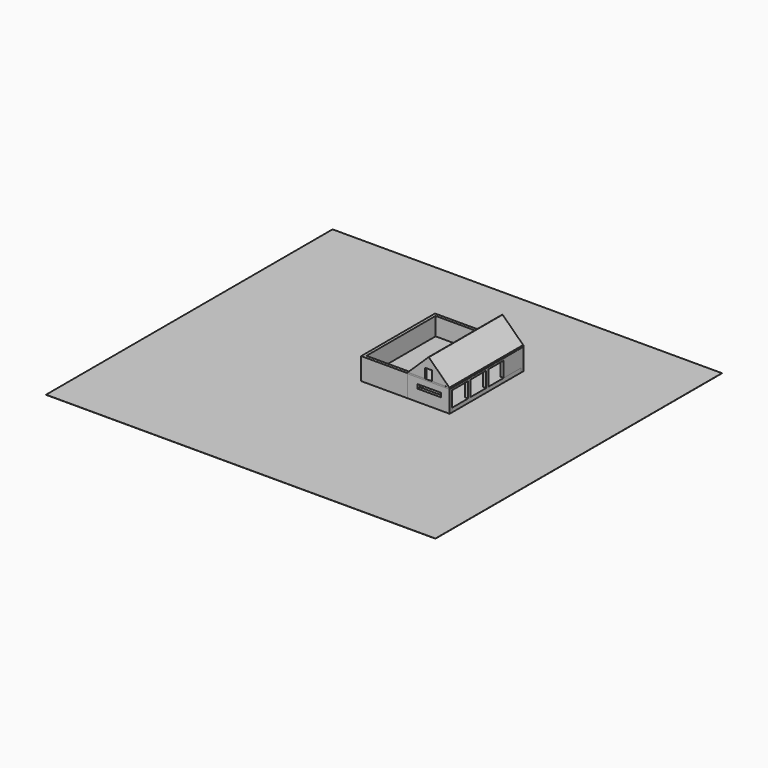
from build123d import *

# Parameters (mm, degrees)
F0_W      = 520
F0_H      = 3240
F0_H_2    = 520
F0_H_3    = 3380
F0_H_4    = 3450
F1_DEPTH  = 10
F2_DEPTH  = 3350
F3_W      = 520
F3_H      = 11110
F4_DEPTH  = 350
F5_W      = 7240
F5_H      = 200
F6_DEPTH  = 200
F7_W      = 7240
F7_H      = 15890
F8_DEPTH  = 3500
F9_SIZE2  = 3499.99999
F9_SIZE   = 3599.99999
F10_T     = 260
F11_W     = 1200
F11_H     = 1700
F12_DEPTH = 260
F13_W     = 6720
F13_H     = 14850
F14_DEPTH = 700
F15_W     = 7240
F15_H     = 15891
F16_DEPTH = 50
F17_W     = 1500
F17_H     = 2650
F18_DEPTH = 520
F19_W     = 4000
F19_H     = 700
F20_DEPTH = 520
F21_W     = 67073.4691619873
F21_H     = 61686.4318847656
F21_W_2   = 7240
F21_H_2   = 15890
F22_DEPTH = 25
F24_DEPTH = 3800
F25_W     = 7500
F25_H     = 14890
F26_DEPTH = 700


# Not quite as in the source:
# - a fillet or chamfer is up to 0.001 mm smaller than in the source, because OpenCascade refuses the exact size
# - a shell that OpenCascade refuses in one call is made with other operations: the cavity is built on its own and cut out
# - a feature names something its author has since deleted; it is built from what else it names


with BuildPart() as f1:
    # F0 (on Top) → F1 (new body)
    with BuildSketch(Plane.XY):
        Polygon((-3374.345998764, -8413.8299859681), (-3374.345998764, 6436.1700140319), (2825.654001236, 6436.1700140319), (2825.654001236, 2696.170014032), (3345.654001236, 2696.170014032), (3345.654001236, 6956.1700140319), (-3894.345998764, 6956.1700140319), (-3894.345998764, -8933.8299859681), (3345.654001236, -8933.8299859681), (3345.654001236, -8413.8299859681), (2825.654001236, -8413.8299859681), align=None)
        Polygon((2825.654001236, 6436.1700140319), (-3374.345998764, 6436.1700140319), (-3374.345998764, -8413.8299859681), (2825.654001236, -8413.8299859681), (2825.654001236, -4963.8299859681), (2825.654001236, -4443.829985968), (2825.654001236, -1063.8299859681), (2825.654001236, -543.829985968), (2825.654001236, 2696.170014032), align=None)
        with Locations((3085.654001236, 1076.170014032)):
            Rectangle(F0_W, F0_H)
        with Locations((3085.654001236, -803.829985968)):
            Rectangle(F0_W, F0_H_2)
        with Locations((3085.654001236, -2753.829985968)):
            Rectangle(F0_W, F0_H_3)
        with Locations((3085.654001236, -6688.8299859681)):
            Rectangle(F0_W, F0_H_4)
        with Locations((3085.654001236, -4703.8299859681)):
            Rectangle(F0_W, F0_H_2)
    extrude(amount=-F1_DEPTH)

    # F0 (on Top) → F2 (join)
    with BuildSketch(Plane.XY):
        with Locations((3085.654001236, -803.829985968)):
            Rectangle(F0_W, F0_H_2)
        with Locations((3085.654001236, -4703.8299859681)):
            Rectangle(F0_W, F0_H_2)
        Polygon((-3374.345998764, -8413.8299859681), (-3374.345998764, 6436.1700140319), (2825.654001236, 6436.1700140319), (2825.654001236, 2696.170014032), (3345.654001236, 2696.170014032), (3345.654001236, 6956.1700140319), (-3894.345998764, 6956.1700140319), (-3894.345998764, -8933.8299859681), (3345.654001236, -8933.8299859681), (3345.654001236, -8413.8299859681), (2825.654001236, -8413.8299859681), align=None)
    extrude(amount=F2_DEPTH)

    # F3 (on face) → F4 (join)
    with BuildSketch(Plane.XY.offset(3350)):
        Polygon((3345.654001236, 6956.1700140319), (-3894.345998764, 6956.1700140319), (-3894.345998764, -8933.8299859681), (3345.654001236, -8933.8299859681), (3345.654001236, -8413.8299859681), (2825.654001236, -8413.8299859681), (-3374.345998764, -8413.8299859681), (-3374.345998764, 6436.1700140319), (2825.654001236, 6436.1700140319), (2825.654001236, 2696.170014032), (3345.654001236, 2696.170014032), align=None)
        with Locations((3085.654001236, -2858.8299859681)):
            Rectangle(F3_W, F3_H)
    extrude(amount=F4_DEPTH)

    # F5 (on face) → F6 (join)
    with BuildSketch(Plane.XY.offset(3700)):
        with Locations((-274.345998764, 6856.1700140319)):
            Rectangle(F5_W, F5_H)
        with Locations((-274.345998764, 5649.1700140319)):
            Rectangle(F5_W, F5_H)
        with Locations((-274.345998764, 4442.1700140319)):
            Rectangle(F5_W, F5_H)
        with Locations((-274.345998764, 3235.1700140319)):
            Rectangle(F5_W, F5_H)
        with Locations((-274.345998764, 2028.1700140319)):
            Rectangle(F5_W, F5_H)
        with Locations((-274.345998764, 821.1700140319)):
            Rectangle(F5_W, F5_H)
        with Locations((-274.345998764, -385.8299859681)):
            Rectangle(F5_W, F5_H)
        with Locations((-274.345998764, -1592.8299859681)):
            Rectangle(F5_W, F5_H)
        with Locations((-274.345998764, -2799.8299859681)):
            Rectangle(F5_W, F5_H)
        with Locations((-274.345998764, -4006.8299859681)):
            Rectangle(F5_W, F5_H)
        with Locations((-274.345998764, -5213.8299859681)):
            Rectangle(F5_W, F5_H)
        with Locations((-274.345998764, -6420.8299859681)):
            Rectangle(F5_W, F5_H)
        with Locations((-274.345998764, -7627.8299859681)):
            Rectangle(F5_W, F5_H)
        with Locations((-274.345998764, -8834.8299859681)):
            Rectangle(F5_W, F5_H)
    extrude(amount=F6_DEPTH)

    # F17 (on face) → F18 (cut)
    with BuildSketch(Plane(origin=(-3894.345998764, 0, 0), x_dir=(0, -1, 0), z_dir=(-1, 0, 0))):
        with Locations((5683.8299859681, 2025)):
            Rectangle(F17_W, F17_H)
        with Locations((1683.8299859681, 2025)):
            Rectangle(F17_W, F17_H)
        with Locations((-2316.1700140319, 2025)):
            Rectangle(F17_W, F17_H)
    extrude(amount=-F18_DEPTH, mode=Mode.SUBTRACT)

    # F19 (on face) → F20 (cut)
    with BuildSketch(Plane.XZ.offset(8933.8299859681)):
        with Locations((-154.345998764, 2350)):
            Rectangle(F19_W, F19_H)
    extrude(amount=-F20_DEPTH, mode=Mode.SUBTRACT)


with BuildPart() as f8:
    # F7 (on face) → F8 (new body)
    with BuildSketch(Plane.XY.offset(3900)):
        with Locations((-274.345998764, -988.8299859681)):
            Rectangle(F7_W, F7_H)
    extrude(amount=F8_DEPTH)

    # F9 (size 3600 and 3500 in the source; OpenCascade refuses exactly that, so slightly less here)
    f9_edges = [f8.edges().sort_by_distance(p)[0] for p in [
        (-3894.345999, -988.829986, 7400),
        (3345.654001, -988.829986, 7400),
    ]]
    f9_side = f8.faces().sort_by_distance((-274.345999, -988.829986, 7400))[0]
    chamfer(f9_edges, length=F9_SIZE, length2=F9_SIZE2, reference=f9_side)

    # F10: shell of thickness 260, made by hand


with BuildPart() as f10_core1:
    # F10_t2: copy of F8
    add(f8.part)

    # the walls: a layer under each face that stays
    f10_faces = [f10_core1.faces().sort_by_distance(p)[0] for p in [
        (-274.3459987642, -8933.8299859681, 5650.0000000001),
        (-3894.345998764, -988.8299859681, 3900.0000050002),
        (-2094.3460037642, -988.8299859681, 5650.0000050002),
        (-274.345998764, -988.8299859681, 7400),
        (3345.654001236, -988.8299859681, 3900.0000050002),
        (1545.6540062361, -988.8299859681, 5650.0000050002),
        (-274.3459987639, 6956.1700140319, 5650.0000000001),
    ]]
    thicken(f10_faces, amount=-F10_T, mode=Mode.SUBTRACT)


with BuildPart() as f8_1:
    add(f8.part)

    # what is left inside the walls is the cavity
    f10_cavity = [f10_core1.part.solids().sort_by_distance(p)[0] for p in [
        (-274.345999, -3550.496653, 3902.6),
    ]]
    add(f10_cavity, mode=Mode.SUBTRACT)

    # F11 (on face) → F12 (cut)
    with BuildSketch(Plane.XZ.offset(8933.8299859681)):
        with Locations((-274.345998764, 4750)):
            Rectangle(F11_W, F11_H)
    extrude(amount=-F12_DEPTH, mode=Mode.SUBTRACT)


with BuildPart() as f14:
    # F13 (on face) → F14 (new body)
    with BuildSketch(Plane.XY):
        with Locations((-14.345998764, -988.8299859681)):
            Rectangle(F13_W, F13_H)
    extrude(amount=F14_DEPTH)


with BuildPart() as f16:
    # F15 (on face) → F16 (new body)
    with BuildSketch(Plane.XY.offset(3900)):
        with Locations((-274.345998764, -989.3299859681)):
            Rectangle(F15_W, F15_H)
    extrude(amount=F16_DEPTH)


with BuildPart() as f22:
    # F21 (on face) → F22 (new body)
    with BuildSketch(Plane(origin=(0, 0, -10), x_dir=(1, 0, 0), z_dir=(0, 0, -1))):
        with Locations((-8991.9595718384, 7652.2979736328)):
            Rectangle(F21_W, F21_H)
        with Locations((-274.345998764, 988.8299859681)):
            Rectangle(F21_W_2, F21_H_2, mode=Mode.SUBTRACT)
    extrude(amount=F22_DEPTH)


with BuildPart() as f24:
    # F23 (on face) → F24 (new body)
    with BuildSketch(Plane.XY.offset(-10)):
        Polygon((-3894.345998764, 6456.1700140319), (-3894.345998764, 6956.1700140319), (-11894.345998764, 6956.1700140319), (-11894.345998764, -8933.8299859681), (-3894.345998764, -8933.8299859681), (-3894.345998764, -8433.8299859681), (-11394.345998764, -8433.8299859681), (-11394.345998764, 6456.1700140319), align=None)
    extrude(amount=F24_DEPTH)


with BuildPart() as f26:
    # F25 (on face) → F26 (new body)
    with BuildSketch(Plane.XY.offset(-10)):
        with Locations((-7644.345998764, -988.8299859681)):
            Rectangle(F25_W, F25_H)
    extrude(amount=F26_DEPTH)


solid = Compound([f1.part, f8_1.part, f14.part, f16.part, f22.part, f24.part, f26.part])
